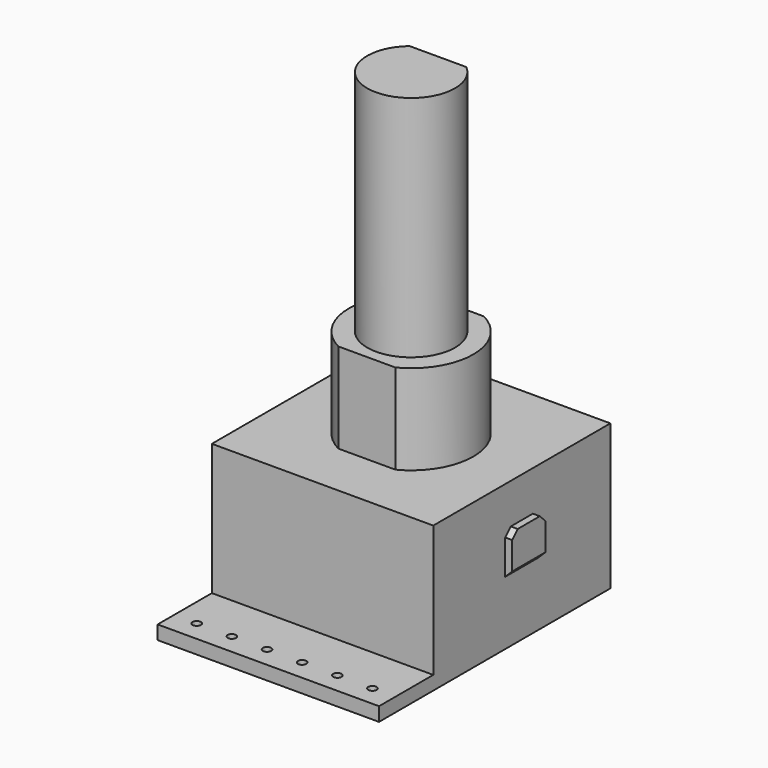
from build123d import *

# Parameters (mm, degrees)
F0_W      = 16
F0_H      = 20.9
F1_DEPTH  = 1
F2_W      = 16
F2_H      = 16
F3_DEPTH  = 9.5
F5_DEPTH  = 6.5
F6_R      = 3.175
F7_DEPTH  = 16.5
F9_DEPTH  = 14
F10_R     = 0.3
F11_DEPTH = 1
F12_W     = 3
F12_H     = 3
F13_DEPTH = 0.5
F14_W     = 3
F14_H     = 3
F15_DEPTH = 0.5
F16_SIZE  = 0.5
F17_SIZE  = 0.49999
F18_SIZE  = 0.49999
F19_SIZE  = 0.5


# Not quite as in the source:
# - a fillet or chamfer is up to 0.001 mm smaller than in the source, because OpenCascade refuses the exact size


with BuildPart() as f1:
    # F0 (on Top) → F1 (new body)
    with BuildSketch(Plane.XY):
        with Locations((0, -2.45)):
            Rectangle(F0_W, F0_H)
    extrude(amount=F1_DEPTH)

    # F2 (on face) → F3 (join)
    with BuildSketch(Plane.XY.offset(1)):
        Rectangle(F2_W, F2_H)
    extrude(amount=F3_DEPTH)

    # F4 (on face) → F5 (join)
    with BuildSketch(Plane.XY.offset(10.5)):
        with BuildLine():
            Line((2.0615528128, 4), (-2.0615528128, 4))
            ThreePointArc((-2.0615528128, 4), (-4.5, 0), (-2.0615528128, -4))
            Line((-2.0615528128, -4), (2.0615528128, -4))
            ThreePointArc((2.0615528128, -4), (4.5, 0), (2.0615528128, 4))
        make_face()
    extrude(amount=F5_DEPTH)

    # F6 (on face) → F7 (join)
    with BuildSketch(Plane.XY.offset(17)):
        Circle(F6_R)
    extrude(amount=F7_DEPTH)

    # F8 (on face) → F9 (cut)
    with BuildSketch(Plane.XY.offset(33.5)):
        with BuildLine():
            ThreePointArc((2.0493901532, 2.425), (0, 3.175), (-2.0493901532, 2.425))
            Line((-2.0493901532, 2.425), (2.0493901532, 2.425))
        make_face()
    extrude(amount=-F9_DEPTH, mode=Mode.SUBTRACT)

    # F10 (on face) → F11 (cut, through all)
    with BuildSketch(Plane(origin=(0, 0, 0), x_dir=(1, 0, 0), z_dir=(0, 0, -1))):
        with Locations((-6.35, 11.43)):
            Circle(F10_R)
        with Locations((-3.81, 11.43)):
            Circle(F10_R)
        with Locations((-1.27, 11.43)):
            Circle(F10_R)
        with Locations((1.27, 11.43)):
            Circle(F10_R)
        with Locations((3.81, 11.43)):
            Circle(F10_R)
        with Locations((6.35, 11.43)):
            Circle(F10_R)
    extrude(amount=-F11_DEPTH, mode=Mode.SUBTRACT)

    # F12 (on face) → F13 (join)
    with BuildSketch(Plane(origin=(-8, 0, 0), x_dir=(0, -1, 0), z_dir=(-1, 0, 0))):
        with Locations((0, 6.1)):
            Rectangle(F12_W, F12_H)
    extrude(amount=F13_DEPTH)

    # F14 (on face) → F15 (join)
    with BuildSketch(Plane.YZ.offset(8)):
        with Locations((0, 6.1)):
            Rectangle(F14_W, F14_H)
    extrude(amount=F15_DEPTH)

    # F16
    f16_edges = [f1.edges().sort_by_distance(p)[0] for p in [
        (-8.25, 1.5, 7.6),
        (-8.25, -1.5, 7.6),
    ]]
    chamfer(f16_edges, length=F16_SIZE)

    # F17 (size 0.5 in the source; OpenCascade refuses exactly that, so slightly less here)
    f17_edges = [f1.edges().sort_by_distance(p)[0] for p in [
        (-8.5, 0, 4.6),
    ]]
    chamfer(f17_edges, length=F17_SIZE)

    # F18 (size 0.5 in the source; OpenCascade refuses exactly that, so slightly less here)
    f18_edges = [f1.edges().sort_by_distance(p)[0] for p in [
        (8.5, 0, 4.6),
    ]]
    chamfer(f18_edges, length=F18_SIZE)

    # F19
    f19_edges = [f1.edges().sort_by_distance(p)[0] for p in [
        (8.25, 1.5, 7.6),
        (8.25, -1.5, 7.6),
    ]]
    chamfer(f19_edges, length=F19_SIZE)


solid = f1.part
